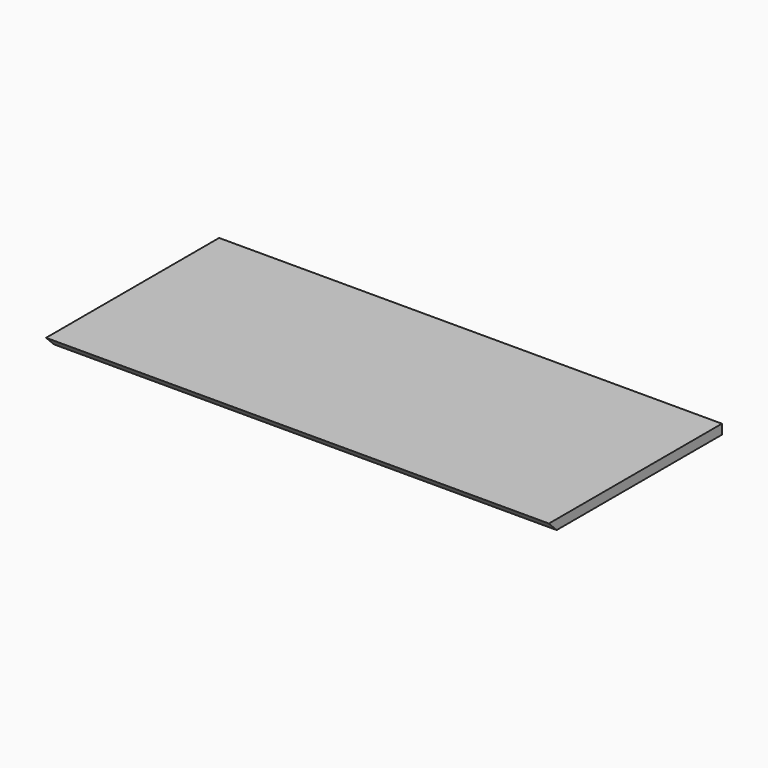
from build123d import *

# Parameters (mm, degrees)
F0_W     = 930
F0_H     = 400
F1_DEPTH = 18
F2_SIZE  = 17.99999


# Not quite as in the source:
# - a fillet or chamfer is up to 0.001 mm smaller than in the source, because OpenCascade refuses the exact size


with BuildPart() as f1:
    # F0 (on Top) → F1 (new body)
    with BuildSketch(Plane.XY):
        Rectangle(F0_W, F0_H)
    extrude(amount=-F1_DEPTH)

    # F2 (size 18 in the source; OpenCascade refuses exactly that, so slightly less here)
    f2_edges = [f1.edges().sort_by_distance(p)[0] for p in [
        (0, -200, -18),
    ]]
    chamfer(f2_edges, length=F2_SIZE)


solid = f1.part
